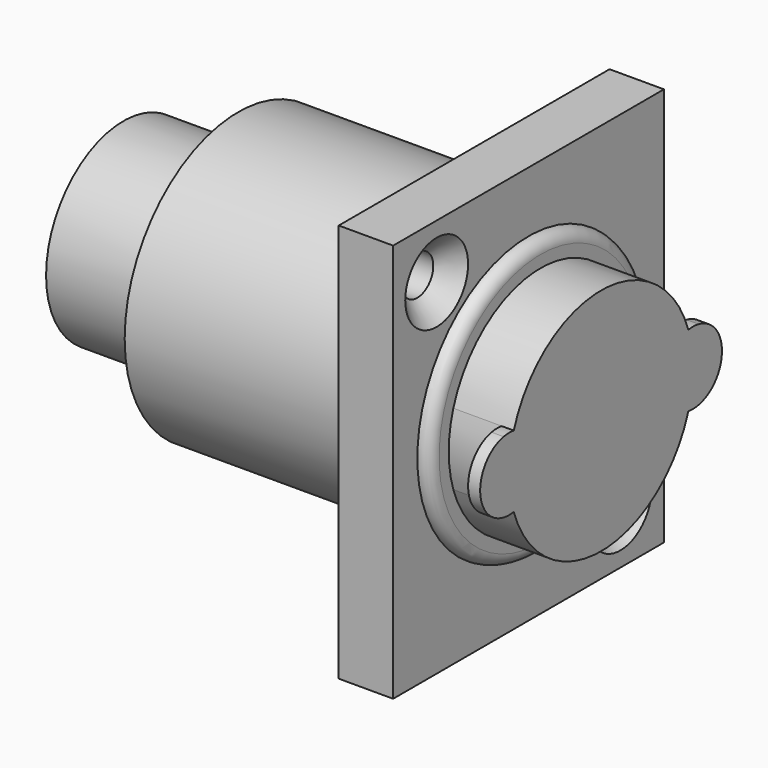
from build123d import *
from build123d import SkipClean  # not in build123d's __all__

# Parameters (mm, degrees)
F0_W            = 28
F0_H            = 33
F1_DEPTH        = 4.5
F2_R            = 11.7475
F3_DEPTH        = 20
F4_R            = 8
F5_DEPTH        = 9.5
F6_R            = 11.5
F7_DEPTH        = 1
F8_R            = 0.99999
F10_DEPTH       = 5
F11_DEPTH       = 4
F13_D           = 3.3
F13_CSINK_D     = 6.5
F13_CSINK_ANGLE = 90
F14_D           = 3.3
F14_CSINK_D     = 6.5
F14_CSINK_ANGLE = 90


# Not quite as in the source:
# - a fillet or chamfer is up to 0.001 mm smaller than in the source, because OpenCascade refuses the exact size


with BuildPart() as f1:
    # F0 (on Right) → F1 (new body)
    with BuildSketch(Plane.YZ):
        with Locations((14, -16.5)):
            Rectangle(F0_W, F0_H)
    extrude(amount=F1_DEPTH)

    # F6 (on face) → F7 (join)
    with BuildSketch(Plane.YZ.offset(4.5)):
        with Locations((14, -16.5)):
            Circle(F6_R)
    extrude(amount=F7_DEPTH)

    # F8 (radius 1 in the source; OpenCascade refuses exactly that, so slightly less here)
    f8_edges = [f1.edges().sort_by_distance(p)[0] for p in [
        (5.5, 2.5, -16.5),
    ]]
    fillet(f8_edges, radius=F8_R)

    # F13 (through all)
    with Locations(Plane.YZ.offset(4.5)):
        with Locations((4.5, -4.5)):
            CounterSinkHole(F13_D / 2, F13_CSINK_D / 2, counter_sink_angle=F13_CSINK_ANGLE)

    # F14 (through all)
    with Locations(Plane.YZ.offset(4.5)):
        with Locations((23.5, -28.5)):
            CounterSinkHole(F14_D / 2, F14_CSINK_D / 2, counter_sink_angle=F14_CSINK_ANGLE)


with BuildPart() as f3:
    # F2 (on face) → F3 (new body)
    with BuildSketch(Plane(origin=(0, 0, 0), x_dir=(0, -1, 0), z_dir=(-1, 0, 0))):
        with Locations((-14.6148139611, -15.9219913185)):
            Circle(F2_R)
    extrude(amount=F3_DEPTH)

    # F4 (on face) → F5 (join)
    with BuildSketch(Plane(origin=(-20, 0, 0), x_dir=(0, -1, 0), z_dir=(-1, 0, 0))):
        with Locations((-14.6148139611, -15.9219913185)):
            Circle(F4_R)
    extrude(amount=F5_DEPTH)


with BuildPart() as f10:
    # F9 (on face) → F10 (new body)
    with BuildSketch(Plane.YZ.offset(5.5)):
        with BuildLine():
            ThreePointArc((4.9736842105, -13.5376321517), (4.5, -16.5), (4.9736842105, -19.4623678483))
            ThreePointArc((4.9736842105, -19.4623678483), (14, -26), (23.0263157895, -19.4623678483))
            ThreePointArc((23.0263157895, -19.4623678483), (23.5, -16.5), (23.0263157895, -13.5376321517))
            ThreePointArc((23.0263157895, -13.5376321517), (14, -7), (4.9736842105, -13.5376321517))
        make_face()
        with BuildLine():
            ThreePointArc((3.9210415789, -13.5563955519), (1.5, -16.5), (3.9210415789, -19.4436044481))
            ThreePointArc((3.9210415789, -19.4436044481), (3.49999, -16.5), (3.9210415789, -13.5563955519))
        make_face()
        with BuildLine():
            ThreePointArc((24.50001, -16.5), (24.3942141168, -17.9867827329), (24.0789584211, -19.4436044481))
            ThreePointArc((24.0789584211, -19.4436044481), (26.5, -16.5), (24.0789584211, -13.5563955519))
            ThreePointArc((24.0789584211, -13.5563955519), (24.3942141168, -15.0132172671), (24.50001, -16.5))
        make_face()
        with BuildLine():
            ThreePointArc((3.9210415789, -19.4436044481), (4.4465333642, -19.4995235153), (4.9736842105, -19.4623678483))
            ThreePointArc((4.9736842105, -19.4623678483), (4.5, -16.5), (4.9736842105, -13.5376321517))
            ThreePointArc((4.9736842105, -13.5376321517), (4.4465333642, -13.5004764847), (3.9210415789, -13.5563955519))
            ThreePointArc((3.9210415789, -13.5563955519), (3.49999, -16.5), (3.9210415789, -19.4436044481))
        make_face()
        with BuildLine():
            ThreePointArc((23.0263157895, -13.5376321517), (23.5, -16.5), (23.0263157895, -19.4623678483))
            ThreePointArc((23.0263157895, -19.4623678483), (23.5534666358, -19.4995235153), (24.0789584211, -19.4436044481))
            ThreePointArc((24.0789584211, -19.4436044481), (24.3942141168, -17.9867827329), (24.50001, -16.5))
            ThreePointArc((24.50001, -16.5), (24.3942141168, -15.0132172671), (24.0789584211, -13.5563955519))
            ThreePointArc((24.0789584211, -13.5563955519), (23.5534666358, -13.5004764847), (23.0263157895, -13.5376321517))
        make_face()
    extrude(amount=F10_DEPTH)

    # F9 (on face) → F11 (cut)
    with BuildSketch(Plane.YZ.offset(5.5)):
        with BuildLine():
            ThreePointArc((3.9210415789, -19.4436044481), (4.4465333642, -19.4995235153), (4.9736842105, -19.4623678483))
            ThreePointArc((4.9736842105, -19.4623678483), (4.5, -16.5), (4.9736842105, -13.5376321517))
            ThreePointArc((4.9736842105, -13.5376321517), (4.4465333642, -13.5004764847), (3.9210415789, -13.5563955519))
            ThreePointArc((3.9210415789, -13.5563955519), (3.49999, -16.5), (3.9210415789, -19.4436044481))
        make_face()
        with BuildLine():
            ThreePointArc((3.9210415789, -13.5563955519), (1.5, -16.5), (3.9210415789, -19.4436044481))
            ThreePointArc((3.9210415789, -19.4436044481), (3.49999, -16.5), (3.9210415789, -13.5563955519))
        make_face()
        with BuildLine():
            ThreePointArc((23.0263157895, -13.5376321517), (23.5, -16.5), (23.0263157895, -19.4623678483))
            ThreePointArc((23.0263157895, -19.4623678483), (23.5534666358, -19.4995235153), (24.0789584211, -19.4436044481))
            ThreePointArc((24.0789584211, -19.4436044481), (24.3942141168, -17.9867827329), (24.50001, -16.5))
            ThreePointArc((24.50001, -16.5), (24.3942141168, -15.0132172671), (24.0789584211, -13.5563955519))
            ThreePointArc((24.0789584211, -13.5563955519), (23.5534666358, -13.5004764847), (23.0263157895, -13.5376321517))
        make_face()
        with BuildLine():
            ThreePointArc((24.50001, -16.5), (24.3942141168, -17.9867827329), (24.0789584211, -19.4436044481))
            ThreePointArc((24.0789584211, -19.4436044481), (26.5, -16.5), (24.0789584211, -13.5563955519))
            ThreePointArc((24.0789584211, -13.5563955519), (24.3942141168, -15.0132172671), (24.50001, -16.5))
        make_face()
    with SkipClean():  # cleaning this boolean's faces spoils the solid; the shape is the same uncleaned
        extrude(amount=F11_DEPTH, mode=Mode.SUBTRACT)


solid = Compound([f1.part, f3.part, f10.part])
